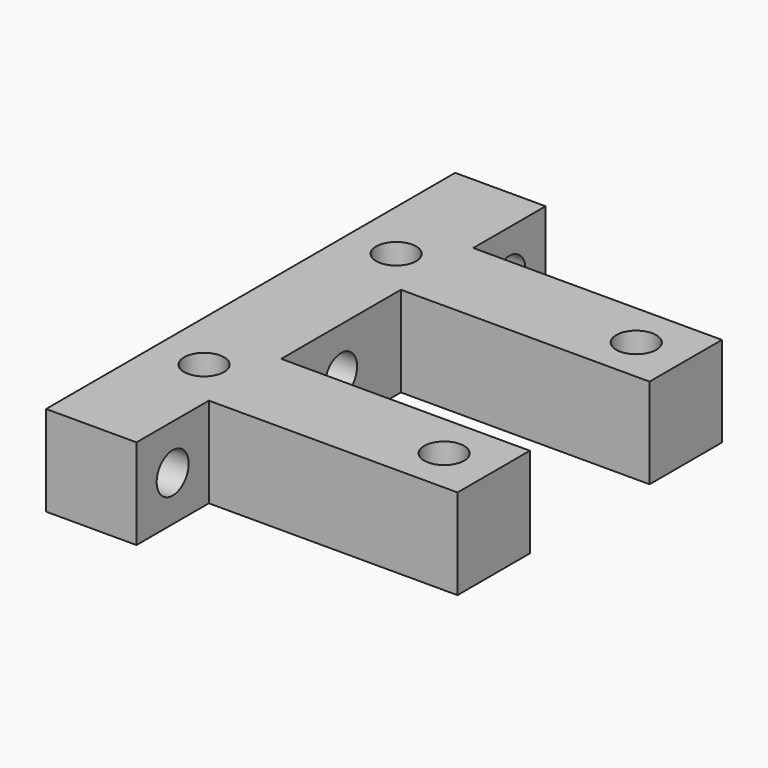
from build123d import *

# Parameters (mm, degrees)
F0_W     = 10.16
F0_H     = 10.16
F0_W_2   = 27.94
F1_DEPTH = 10.16
F2_D     = 4.4958
F3_D     = 4.4958
F4_D     = 4.4958
F5_D     = 4.4958
F7_D     = 4.4958
F10_D    = 4.4958
F11_D    = 4.4958


# Not quite as in the source:
# - a feature names something its author has since deleted; it is built from what else it names


with BuildPart() as f1:
    # F0 (on Top) → F1 (new body)
    with BuildSketch(Plane.XY):
        Polygon((-19.05, 32.0548), (-19.05, -5.08), (-8.89, -5.08), (-8.89, 5.08), (-8.89, 21.8948), (-8.89, 32.0548), align=None)
        with Locations((-13.97, -10.16)):
            Rectangle(F0_W, F0_H)
        with Locations((5.08, 0)):
            Rectangle(F0_W_2, F0_H)
        with Locations((-13.97, 37.1348)):
            Rectangle(F0_W, F0_H)
        with Locations((5.08, 26.9748)):
            Rectangle(F0_W_2, F0_H)
    extrude(amount=F1_DEPTH)

    # F2 (through all)
    with Locations(Plane(origin=(0, 0, 0), x_dir=(1, 0, 0), z_dir=(0, 0, -1))):
        with Locations((13.4874, 0)):
            Hole(F2_D / 2)

    # F3 (through all)
    with Locations(Plane(origin=(0, 0, 0), x_dir=(1, 0, 0), z_dir=(0, 0, -1))):
        with Locations((-13.4874, 0)):
            Hole(F3_D / 2)

    # F4 (through all)
    with Locations(Plane(origin=(0, 0, 0), x_dir=(1, 0, 0), z_dir=(0, 0, -1))):
        with Locations((-13.4874, -26.9748)):
            Hole(F4_D / 2)

    # F5 (through all)
    with Locations(Plane(origin=(0, 0, 0), x_dir=(1, 0, 0), z_dir=(0, 0, -1))):
        with Locations((13.4874, -26.9748)):
            Hole(F5_D / 2)

    # F7 (through all)
    with Locations(Plane.YZ.offset(-8.89)):
        with Locations((13.4874, 5.08)):
            Hole(F7_D / 2)

    # F10 (through all)
    with Locations(Plane.YZ.offset(-8.89)):
        with Locations((-10.16, 5.08)):
            Hole(F10_D / 2)

    # F11 (through all)
    with Locations(Plane.YZ.offset(-8.89)):
        with Locations((37.1348, 5.08)):
            Hole(F11_D / 2)


solid = f1.part
